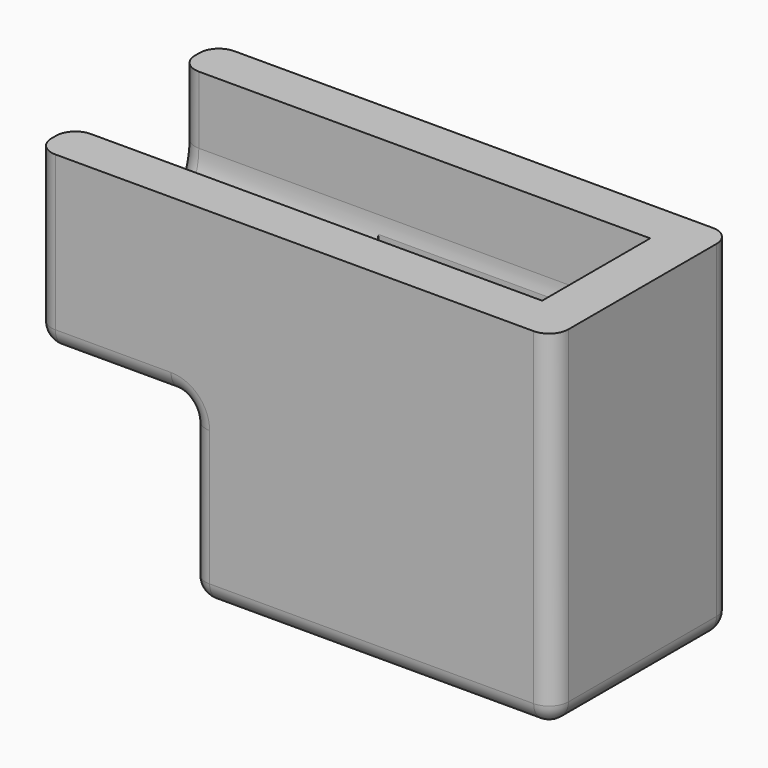
from build123d import *

# Parameters (mm, degrees)
F0_W     = 4
F0_H     = 5.8
F0_W_2   = 9.4
F0_W_3   = 7
F0_H_2   = 3.4
F1_DEPTH = 9
F2_DEPTH = 4.5
F4_DEPTH = 12.2
F5_R     = 0.49999


# Not quite as in the source:
# - a fillet or chamfer is up to 0.001 mm smaller than in the source, because OpenCascade refuses the exact size


with BuildPart() as f1:
    # F0 (on Top) → F1 (new body)
    with BuildSketch(Plane.XY):
        with Locations((-6.7, 0)):
            Rectangle(F0_W, F0_H)
        Rectangle(F0_W_2, F0_H)
        Rectangle(F0_W_3, F0_H_2, mode=Mode.SUBTRACT)
    extrude(amount=F1_DEPTH)

    # F0 (on Top) → F2 (cut)
    with BuildSketch(Plane.XY):
        with Locations((-6.7, 0)):
            Rectangle(F0_W, F0_H)
    extrude(amount=F2_DEPTH, mode=Mode.SUBTRACT)

    # F3 (on face) → F4 (cut, through all)
    with BuildSketch(Plane(origin=(-8.7, 0, 0), x_dir=(0, -1, 0), z_dir=(-1, 0, 0))):
        with BuildLine():
            Line((-1.75, 9), (-1.75, 7.25))
            ThreePointArc((-1.75, 7.25), (0, 5.5), (1.75, 7.25))
            Line((1.75, 7.25), (1.75, 9))
            Line((1.75, 9), (-1.75, 9))
        make_face()
    extrude(amount=-F4_DEPTH, mode=Mode.SUBTRACT)

    # F5 (radius 0.5 in the source; OpenCascade refuses exactly that, so slightly less here)
    f5_edges = [f1.edges().sort_by_distance(p)[0] for p in [
        (-4.7, 2.9, 2.25),
        (-6.7, 2.9, 4.5),
        (-4.7, 0, 4.5),
        (-4.7, -2.9, 2.25),
        (4.7, -2.9, 4.5),
        (4.7, 2.9, 4.5),
        (0, 2.9, 0),
        (4.7, 0, 0),
        (0, -2.9, 0),
        (-4.7, 0, 0),
        (-8.7, 2.9, 6.75),
        (-8.7, 0, 4.5),
        (-8.7, -2.9, 6.75),
        (-8.7, 0, 5.5),
        (-8.7, -1.75, 8.125),
        (-8.7, 1.75, 8.125),
        (-6.7, -2.9, 4.5),
    ]]
    fillet(f5_edges, radius=F5_R)


solid = f1.part
